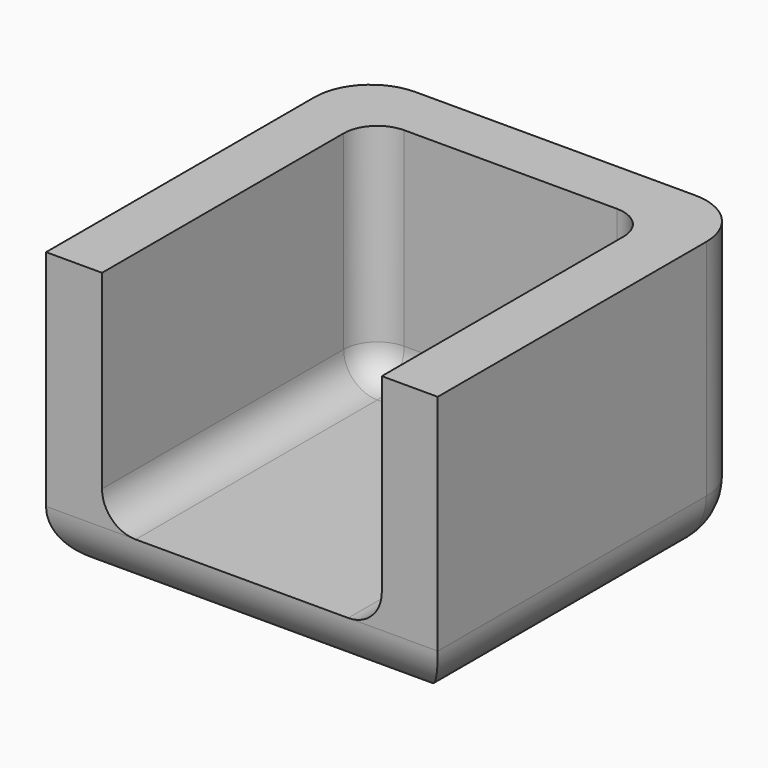
from build123d import *

# Parameters (mm, degrees)
F1_DEPTH = 20
F0_W     = 25
F0_H     = 30
F2_DEPTH = 5
F3_R     = 4.99999
F4_R     = 3


# Not quite as in the source:
# - a fillet or chamfer is up to 0.001 mm smaller than in the source, because OpenCascade refuses the exact size


with BuildPart() as f1:
    # F0 (on Top) → F1 (new body)
    with BuildSketch(Plane.XY):
        with BuildLine():
            Line((12.5, -17.5), (17.5, -17.5))
            Line((17.5, -17.5), (17.5, 12.5))
            ThreePointArc((17.5, 12.5), (16.0355339059, 16.0355339059), (12.5, 17.5))
            Line((12.5, 17.5), (-12.5, 17.5))
            ThreePointArc((-12.5, 17.5), (-16.0355339059, 16.0355339059), (-17.5, 12.5))
            Line((-17.5, 12.5), (-17.5, -17.5))
            Line((-17.5, -17.5), (-12.5, -17.5))
            Line((-12.5, -17.5), (-12.5, 12.5))
            Line((-12.5, 12.5), (12.5, 12.5))
            Line((12.5, 12.5), (12.5, -17.5))
        make_face()
    extrude(amount=F1_DEPTH)

    # F0 (on Top) → F2 (join)
    with BuildSketch(Plane.XY):
        with Locations((0, -2.5)):
            Rectangle(F0_W, F0_H)
        with BuildLine():
            Line((12.5, -17.5), (17.5, -17.5))
            Line((17.5, -17.5), (17.5, 12.5))
            ThreePointArc((17.5, 12.5), (16.0355339059, 16.0355339059), (12.5, 17.5))
            Line((12.5, 17.5), (-12.5, 17.5))
            ThreePointArc((-12.5, 17.5), (-16.0355339059, 16.0355339059), (-17.5, 12.5))
            Line((-17.5, 12.5), (-17.5, -17.5))
            Line((-17.5, -17.5), (-12.5, -17.5))
            Line((-12.5, -17.5), (-12.5, 12.5))
            Line((-12.5, 12.5), (12.5, 12.5))
            Line((12.5, 12.5), (12.5, -17.5))
        make_face()
    extrude(amount=-F2_DEPTH)

    # F3 (radius 5 in the source; OpenCascade refuses exactly that, so slightly less here)
    f3_edges = [f1.edges().sort_by_distance(p)[0] for p in [
        (17.5, -2.5, -5),
        (16.035534, 16.035534, -5),
        (0, 17.5, -5),
        (-16.035534, 16.035534, -5),
        (-17.5, -2.5, -5),
        (0, -17.5, -5),
    ]]
    fillet(f3_edges, radius=F3_R)

    # F4
    f4_edges = [f1.edges().sort_by_distance(p)[0] for p in [
        (12.5, -2.5, 0),
        (-12.5, -2.5, 0),
        (12.5, 12.5, 10),
        (-12.5, 12.5, 10),
        (0, 12.5, 0),
    ]]
    fillet(f4_edges, radius=F4_R)


solid = f1.part
